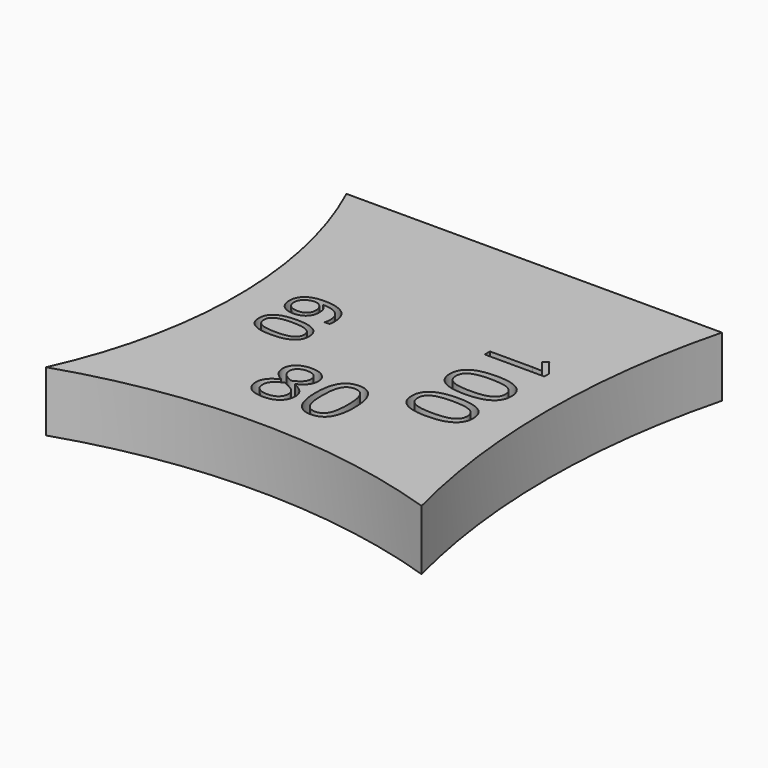
from build123d import *

# Parameters (mm, degrees)
F0_W           = 50
F0_H           = 50
F1_DEPTH       = 8
F2_TEXT_SIZE   = 11.1111111111
F2_TEXT_SIZE_2 = 9.0534126179
F3_DEPTH       = 25
F4_W           = 36.4681230858
F4_H           = 30.478188768
F5_DEPTH       = 2


# Not quite as in the source:
# - Text() gives the source's letters only with a copy of the font that has no kerning and outlines rounded to 1/6400 em; it was checked with that copy


with BuildPart() as f1:
    # F0 (on Top) → F1 (new body)
    with BuildSketch(Plane.XY):
        with Locations((25, -25)):
            Rectangle(F0_W, F0_H)
    extrude(amount=F1_DEPTH)

    # F2 (on face) → F3 (cut)
    with BuildSketch(Plane.XY.offset(8)):
        with BuildLine():
            ThreePointArc((50, -50), (25, -45.9934207679), (0, -50))
            ThreePointArc((0, -50), (5.4564394268, -25), (0, 0))
            Line((0, 0), (-44.3667769432, -1.7646922497))
            Line((-44.3667769432, -1.7646922497), (-30.6636244059, -60.3145584464))
            Line((-30.6636244059, -60.3145584464), (36.1081436276, -65.0483816862))
            Line((36.1081436276, -65.0483816862), (101.6341671348, -49.8503260314))
            Line((101.6341671348, -49.8503260314), (67.0025423169, -23.4406031668))
            Line((67.0025423169, -23.4406031668), (50, 0))
            ThreePointArc((50, 0), (46.8245836552, -25), (50, -50))
        make_face()
        with Locations(Location((33.8245836552, -15.3871527778), (0, 0, -90))):
            Text('100', F2_TEXT_SIZE, font='Open Sans', text_align=(TextAlign.LEFT, TextAlign.BOTTOM))
        with Locations((18.5633680556, -40.9934207679)):
            Text('80', F2_TEXT_SIZE, font='Open Sans', text_align=(TextAlign.LEFT, TextAlign.BOTTOM))
        with Locations(Location((10.4564394268, -19.7553863624), (0, 0, -90))):
            Text('60', F2_TEXT_SIZE_2, font='Open Sans', text_align=(TextAlign.LEFT, TextAlign.BOTTOM))
    extrude(amount=-F3_DEPTH, mode=Mode.SUBTRACT)

    # F4 (on face) → F5 (join)
    with BuildSketch(Plane(origin=(0, 0, 0), x_dir=(1, 0, 0), z_dir=(0, 0, -1))):
        with Locations((26.514263358, 28.5384347662)):
            Rectangle(F4_W, F4_H)
    extrude(amount=-F5_DEPTH)


solid = f1.part
